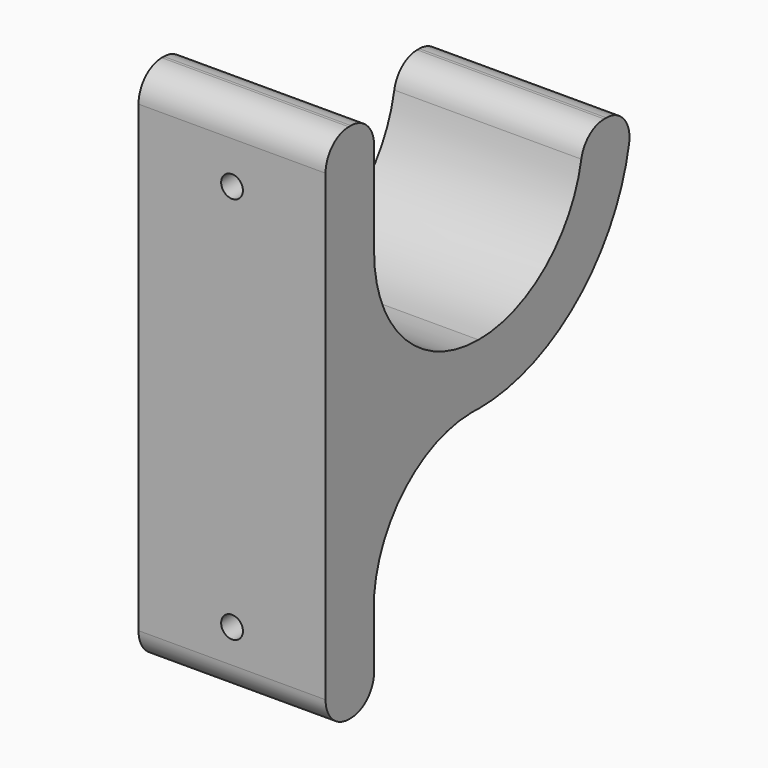
from build123d import *

# Parameters (mm, degrees)
F1_DEPTH       = 58
F2_R           = 9
F4_D           = 6.7564
F4_DEPTH       = 127
F4_CSINK_D     = 13.4874
F4_CSINK_ANGLE = 82
F4_TIP         = 2.0298273432


# Not quite as in the source:
# - a feature names something its author has since deleted; it is built from what else it names


with BuildPart() as f1:
    # F0 (on Right) → F1 (new body)
    with BuildSketch(Plane.YZ):
        with BuildLine():
            Line((59.3103850067, 0), (40.5, 0))
            ThreePointArc((40.5, 0), (28.6378246381, -28.6378246381), (0, -40.5))
            ThreePointArc((0, -40.5), (-28.6378246381, -28.6378246381), (-40.5, 0))
            Line((-40.5, 0), (-40.5, -43.3298023263))
            ThreePointArc((-40.5, -43.3298023263), (-23.1030418264, -54.62573778), (-2.8803521713, -59.2404029443))
            ThreePointArc((-2.8803521713, -59.2404029443), (-1.4395179453, -59.2483059491), (0, -59.3103850067))
            ThreePointArc((0, -59.3103850067), (41.938775433, -41.938775433), (59.3103850067, 0))
        make_face()
        with BuildLine():
            Line((-40.5, -43.3298023263), (-40.5, 0))
            Line((-40.5, 0), (-59.3103850067, 0))
            ThreePointArc((-59.3103850067, 0), (-54.4049279129, -23.6183316184), (-40.5, -43.3298023263))
        make_face()
        with BuildLine():
            Line((-59.3103850067, 0), (-40.5, 0))
            Line((-40.5, 0), (-40.5, 38.1))
            Line((-40.5, 38.1), (-45.4545021933, 38.1))
            ThreePointArc((-45.4545021933, 38.1), (-55.7388813801, 20.2706406444), (-59.3103850067, 0))
        make_face()
        with BuildLine():
            Line((-59.3103850067, 38.1), (-59.3103850067, 0))
            ThreePointArc((-59.3103850067, 0), (-55.7388813801, 20.2706406444), (-45.4545021933, 38.1))
            Line((-45.4545021933, 38.1), (-59.3103850067, 38.1))
        make_face()
        with BuildLine():
            ThreePointArc((-40.5, -43.3298023263), (-54.4049279129, -23.6183316184), (-59.3103850067, 0))
            Line((-59.3103850067, 0), (-59.3103850067, -123.6414313316))
            Line((-59.3103850067, -123.6414313316), (-40.5, -123.6414313316))
            Line((-40.5, -123.6414313316), (-40.5, -93.8428338624))
            Line((-40.5, -93.8428338624), (-40.5, -43.3298023263))
        make_face()
        with BuildLine():
            ThreePointArc((-2.8803521713, -59.2404029443), (-23.1030418264, -54.62573778), (-40.5, -43.3298023263))
            Line((-40.5, -43.3298023263), (-40.5, -93.8428338624))
            ThreePointArc((-40.5, -93.8428338624), (-28.3045630471, -69.3504788941), (-2.8803521713, -59.2404029443))
        make_face()
    extrude(amount=F1_DEPTH)

    # F2
    f2_edges = [f1.edges().sort_by_distance(p)[0] for p in [
        (29, -40.5, 38.1),
        (29, -59.310385, 38.1),
        (29, 59.310385, 0),
        (29, 40.5, 0),
        (29, -40.5, -123.641431),
        (29, -59.310385, -123.641431),
    ]]
    fillet(f2_edges, radius=F2_R)

    # F4
    with Locations(Plane(origin=(0, -40.5, 0), x_dir=(-1, 0, 0), z_dir=(0, 1, 0))):
        with Locations((-29, 16.0360112786), (-29, -104.242132597)):
            CounterSinkHole(F4_D / 2, F4_CSINK_D / 2, depth=F4_DEPTH, counter_sink_angle=F4_CSINK_ANGLE)
            with Locations((0, 0, -(F4_DEPTH + F4_TIP / 2))):  # 118° drill point
                Cone(0, F4_D / 2, F4_TIP, mode=Mode.SUBTRACT)


solid = f1.part
